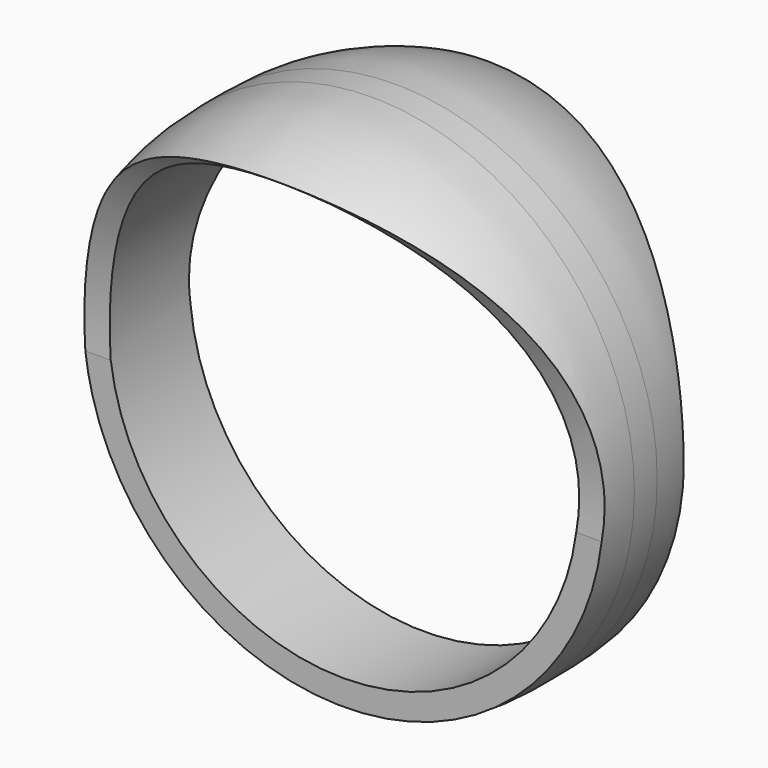
from build123d import *

# Parameters (mm, degrees)
F0_R      = 25
F1_DEPTH  = 25
F2_R      = 22.3658114716
F3_DEPTH  = 32.2
F5_R      = 36.5407800477
F6_DEPTH  = 38.2
F7_R      = 35.8063234998
F8_DEPTH  = 59.2
F10_DEPTH = 36.7
F12_DEPTH = 52.2


# Not quite as in the source:
# - a fillet or chamfer that OpenCascade refuses, or shapes differently, is made with other operations: its cross-section is extruded or revolved along the edge and cut away or added


with BuildPart() as f1:
    # F0 (on Front) → F1 (new body)
    with BuildSketch(Plane.XZ):
        Circle(F0_R)
    extrude(amount=F1_DEPTH)

    # F2 (on face) → F3 (cut, symmetric)
    with BuildSketch(Plane.XZ.offset(25)):
        Circle(F2_R)
    extrude(amount=F3_DEPTH, both=True, mode=Mode.SUBTRACT)

    # F4: fillet of radius 24.8663996924 on 2 edges, made by hand

    # F4_s1 → F4_t2 (revolve, cut)
    with BuildSketch(Plane.XY):
        with BuildLine():
            ThreePointArc((25, -13.8614803309), (24.3324936967, -19.5843635558), (22.3658114716, -25))
            Line((22.3658114716, -25), (22.8104556949, -25.2227703934))
            ThreePointArc((22.8104556949, -25.2227703934), (23.6829057358, -25.4973279938), (25, -25.4973279938))
            Line((25, -25.4973279938), (25.4973279938, -25))
            Line((25.4973279938, -25), (25.4973279938, -13.8614803309))
            Line((25.4973279938, -13.8614803309), (25, -13.8614803309))
        make_face()
    revolve(axis=Axis((0, -25, 0), (0, -1, 0)), mode=Mode.SUBTRACT)

    # F4_s3 → F4_t4 (revolve, cut)
    with BuildSketch(Plane.XY):
        with BuildLine():
            ThreePointArc((25, -11.1385196691), (24.3324936967, -5.4156364442), (22.3658114716, 0))
            Line((22.3658114716, 0), (22.8104556949, 0.2227703934))
            ThreePointArc((22.8104556949, 0.2227703934), (23.6829057358, 0.4973279938), (25, 0.4973279938))
            Line((25, 0.4973279938), (25.4973279938, 0))
            Line((25.4973279938, 0), (25.4973279938, -11.1385196691))
            Line((25.4973279938, -11.1385196691), (25, -11.1385196691))
        make_face()
    revolve(axis=Axis((0, 0, 0), (0, -1, 0)), mode=Mode.SUBTRACT)

    # F5 (on Right) → F6 (cut, symmetric)
    with BuildSketch(Plane.YZ):
        with Locations((28.8398824632, 0)):
            Circle(F5_R)
    extrude(amount=F6_DEPTH, both=True, mode=Mode.SUBTRACT)

    # F7 (on Right) → F8 (cut, symmetric)
    with BuildSketch(Plane.YZ):
        with Locations((-52.9389642179, 0)):
            Circle(F7_R)
    extrude(amount=F8_DEPTH, both=True, mode=Mode.SUBTRACT)

    # F9 (on Right) → F10 (cut, symmetric)
    with BuildSketch(Plane.YZ):
        Polygon((6.057692226, -21.5969905257), (-7.6379603706, 0), (-7.6379603706, -55.3093664348), align=None)
    extrude(amount=F10_DEPTH, both=True, mode=Mode.SUBTRACT)

    # F11 (on Right) → F12 (cut, symmetric)
    with BuildSketch(Plane.YZ):
        Polygon((-17.2512549907, -55.5727444589), (-17.2512549907, 0), (-31.0785956681, -9.4816060737), align=None)
    extrude(amount=F12_DEPTH, both=True, mode=Mode.SUBTRACT)


solid = f1.part
